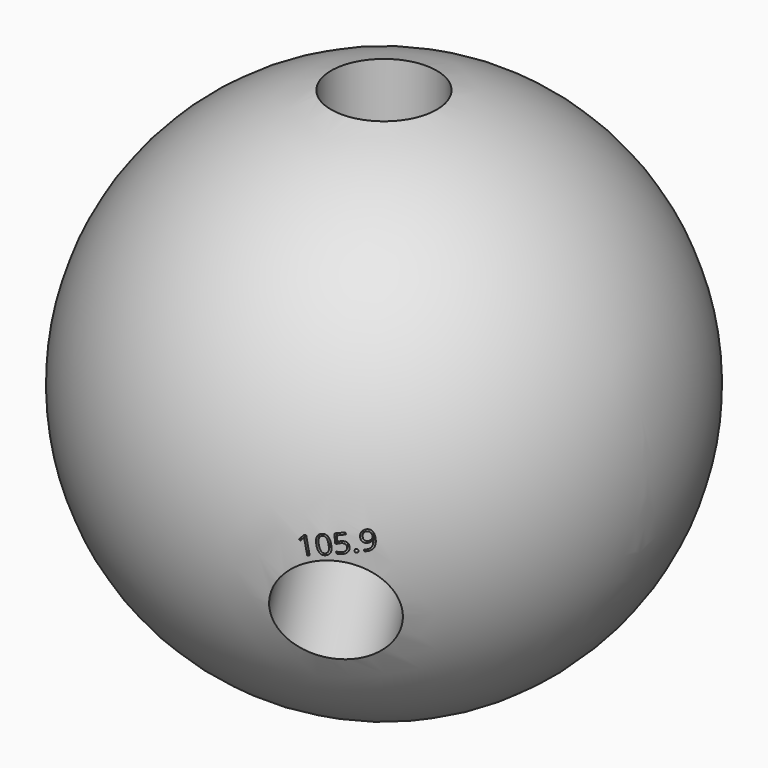
from build123d import *

# Parameters (mm, degrees)
F4_R          = 3.175
F5_DEPTH      = 50.8
F7_ANGLE      = 120
F8_ANGLE      = 109.3
F9_ANGLE      = 120
F10_ANGLE     = -105.9
F11_ANGLE     = -60
F13_TEXT_SIZE = 1.3579025916
F14_DEPTH     = 11.0998
F16_TEXT_SIZE = 1.7828159293
F17_DEPTH     = 4.6228
F19_TEXT_SIZE = 1.5112493808
F20_DEPTH     = 4.4958


# Not quite as in the source:
# - Text() gives the source's letters only with a copy of the font that has no kerning and outlines rounded to 1/6400 em; it was checked with that copy


with BuildPart() as f2:
    # F0 (on Front) → F2 (revolve)
    with BuildSketch(Plane.XZ):
        with BuildLine():
            Line((0, -15.875), (0, 15.875))
            ThreePointArc((0, 15.875), (-15.875, 0), (0, -15.875))
        make_face()
    revolve(axis=Axis((0, 0, 0), (0, 0, 1)))


with BuildPart() as f5:
    # F4 (on offset) → F5 (new body)
    with BuildSketch(Plane.XY.offset(6.35)):
        Circle(F4_R)
    extrude(amount=F5_DEPTH)


with BuildPart() as f7_1:
    # F7: copy of F5
    add(f5.part.rotate(Axis((0, 0, 6.35), (0, 0, -1)), F7_ANGLE))


with BuildPart() as f5_1:
    # F8: moved
    add(f5.part.rotate(Axis((0, -21.7784233391, 0), (0, -1, 0)), F8_ANGLE))


with BuildPart() as f2_1:
    # F8: moved
    add(f2.part.rotate(Axis((0, -21.7784233391, 0), (0, -1, 0)), F8_ANGLE))

    # F13 (on offset) → F14 (cut)
    with BuildSketch(Plane(origin=(-23.9725441702, 0, -8.3950655749), x_dir=(0, -1, 0), z_dir=(-0.9438009516, 0, -0.3305143927))):
        with Locations((-2.0063980483, 3.8888063282)):
            Text('109.3', F13_TEXT_SIZE, font='Open Sans', text_align=(TextAlign.LEFT, TextAlign.BOTTOM))
    extrude(amount=-F14_DEPTH, mode=Mode.SUBTRACT)

    # F16 (on offset) → F17 (cut)
    with BuildSketch(Plane(origin=(8.9897040638, 15.5706241836, -6.2962991812), x_dir=(-0.8816518252, 0.4374861885, -0.1769064553), z_dir=(0.4719004758, 0.8173556002, -0.3305143927))):
        with Locations((-1.7114999937, 3.5567139275)):
            Text('109.3', F16_TEXT_SIZE, font='Open Sans', text_align=(TextAlign.LEFT, TextAlign.BOTTOM))
    extrude(amount=-F17_DEPTH, mode=Mode.SUBTRACT)

    # F19 (on offset) → F20 (cut)
    with BuildSketch(Plane(origin=(9.1605859735, -15.8666003331, -5.2189231161), x_dir=(0.876791545, 0.4567944557, 0.1502511625), z_dir=(0.4808706548, -0.8328924059, -0.2739592187))):
        with Locations((-1.1127216276, 3.4589394927)):
            Text('105.9', F19_TEXT_SIZE, font='Open Sans', text_align=(TextAlign.LEFT, TextAlign.BOTTOM))
    extrude(amount=-F20_DEPTH, mode=Mode.SUBTRACT)


with BuildPart() as f9_1:
    # F9: copy of F5
    add(f5_1.part.rotate(Axis((0, 0, -15.9466937184), (0, 0, -1)), F9_ANGLE))


with BuildPart() as f10_1:
    # F10: copy of F7_1
    add(f7_1.part.rotate(Axis((0, -21.7784233391, 0), (0, -1, 0)), F10_ANGLE))


with BuildPart() as f10_1_1:
    # F11: moved
    add(f10_1.part.rotate(Axis((0, 0, 25.4038926214), (0, 0, 1)), F11_ANGLE))


with BuildPart() as f2_2:
    add(f2_1.part)

    # F21: cut F10_1, F5, F9_1, F7_1
    add(f10_1_1.part, mode=Mode.SUBTRACT)
    add(f5_1.part, mode=Mode.SUBTRACT)
    add(f9_1.part, mode=Mode.SUBTRACT)
    add(f7_1.part, mode=Mode.SUBTRACT)


solid = f2_2.part
